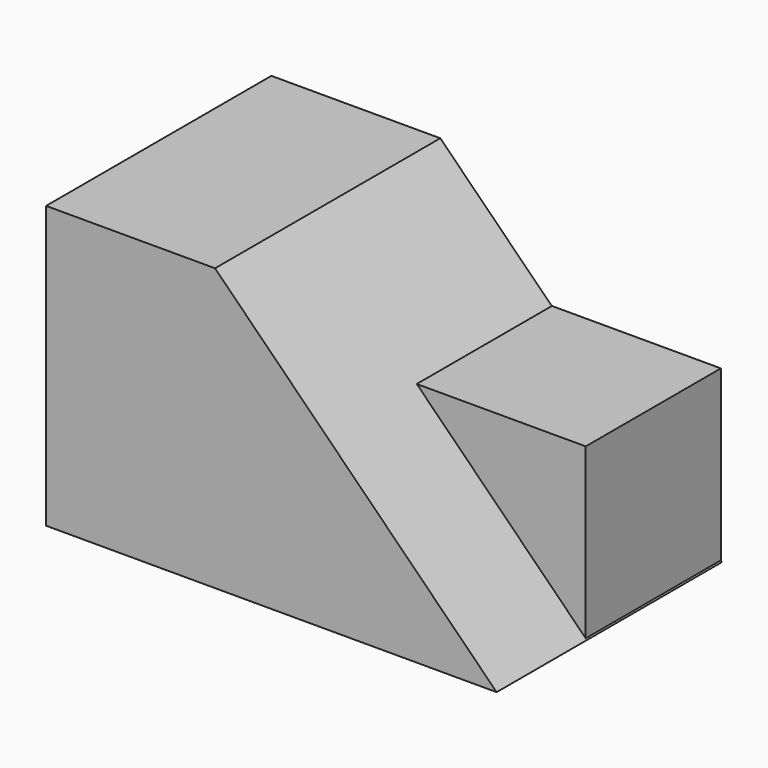
from build123d import *

# Parameters (mm, degrees)
F1_DEPTH = 31.75
F3_DEPTH = 19.05


# Not quite as in the source:
# - a length typed as a fraction of an inch, garbled in the dataset ("3 / 203.2 mm" for 3/8 in), is restored


with BuildPart() as f1:
    # F0 (on Front) → F1 (new body)
    with BuildSketch(Plane.XZ):
        Polygon((-15.9773944168, 34.0396987623), (-35.0273944168, 34.0396987623), (-35.0273944168, 2.2896987623), (15.7726055832, 2.2896987623), align=None)
    extrude(amount=F1_DEPTH)


with BuildPart() as f3:
    # F2 (on Front) → F3 (new body)
    with BuildSketch(Plane.XZ):
        Polygon((-3.3935803209, 21.4862959499), (15.6564196791, 2.436293192), (15.6564196791, 21.4862959499), align=None)
    extrude(amount=F3_DEPTH)


solid = Compound([f1.part, f3.part])
